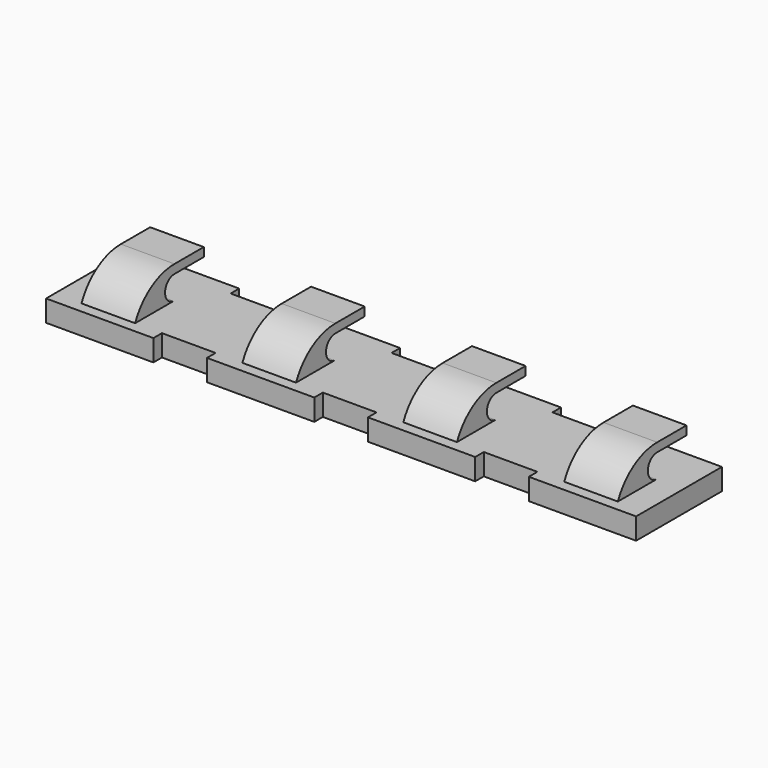
from build123d import *

# Parameters (mm, degrees)
F0_W        = 5
F0_H        = 8
F1_DEPTH    = 2
F2_DEPTH    = 5
F3_T1_DEPTH = 27.9128784748
F3_T3_DEPTH = 27.9128784748
F3_T5_DEPTH = 27.9128784748
F3_T7_DEPTH = 27.9128784748
F5_DEPTH    = 65


# Not quite as in the source:
# - a fillet or chamfer that OpenCascade refuses, or shapes differently, is made with other operations: its cross-section is extruded or revolved along the edge and cut away or added


with BuildPart() as f1:
    # F0 (on Top) → F1 (new body)
    with BuildSketch(Plane.XY):
        Polygon((-17.5, 5), (-27.5, 5), (-27.5, -5), (-17.5, -5), (-17.5, -4), (-17.5, 4), align=None)
        with Locations((-22.5, 0)):
            Rectangle(F0_W, F0_H, mode=Mode.SUBTRACT)
        with Locations((-15, 0)):
            Rectangle(F0_W, F0_H)
        Polygon((-12.5, 5), (-12.5, 4), (-12.5, -4), (-12.5, -5), (-2.5, -5), (-2.5, -4), (-2.5, 4), (-2.5, 5), align=None)
        with Locations((-7.5, 0)):
            Rectangle(F0_W, F0_H, mode=Mode.SUBTRACT)
        Rectangle(F0_W, F0_H)
        Polygon((2.5, 5), (2.5, 4), (2.5, -4), (2.5, -5), (12.5, -5), (12.5, -4), (12.5, 4), (12.5, 5), align=None)
        with Locations((7.5, 0)):
            Rectangle(F0_W, F0_H, mode=Mode.SUBTRACT)
        with Locations((15, 0)):
            Rectangle(F0_W, F0_H)
        Polygon((17.5, 5), (17.5, 4), (17.5, -4), (17.5, -5), (27.5, -5), (27.5, 5), align=None)
        with Locations((22.5, 0)):
            Rectangle(F0_W, F0_H, mode=Mode.SUBTRACT)
    extrude(amount=F1_DEPTH)

    # F0 (on Top) → F2 (join)
    with BuildSketch(Plane.XY):
        with Locations((-22.5, 0)):
            Rectangle(F0_W, F0_H)
        with Locations((-7.5, 0)):
            Rectangle(F0_W, F0_H)
        with Locations((7.5, 0)):
            Rectangle(F0_W, F0_H)
        with Locations((22.5, 0)):
            Rectangle(F0_W, F0_H)
    extrude(amount=F2_DEPTH)

    # F3: fillet of radius 5 on 4 edges, made by hand

    # F3_s2 → F3_t1 (cut)
    with BuildSketch(Plane.YZ.offset(-36.4564392374)):
        with BuildLine():
            ThreePointArc((-4, 2), (-2.1560370926, 4.1833001327), (0.582575695, 5))
            Line((0.582575695, 5), (0.582575695, 5.1))
            Line((0.582575695, 5.1), (-4, 5.1))
            Line((-4, 5.1), (-4.1, 5))
            ThreePointArc((-4.1, 5), (-4.1, 3.5), (-4.0916515139, 2.04))
            Line((-4.0916515139, 2.04), (-4, 2))
        make_face()
    extrude(amount=F3_T1_DEPTH, mode=Mode.SUBTRACT)

    # F3_s4 → F3_t3 (cut)
    with BuildSketch(Plane.YZ.offset(-21.4564392374)):
        with BuildLine():
            ThreePointArc((-4, 2), (-2.1560370926, 4.1833001327), (0.582575695, 5))
            Line((0.582575695, 5), (0.582575695, 5.1))
            Line((0.582575695, 5.1), (-4, 5.1))
            Line((-4, 5.1), (-4.1, 5))
            ThreePointArc((-4.1, 5), (-4.1, 3.5), (-4.0916515139, 2.04))
            Line((-4.0916515139, 2.04), (-4, 2))
        make_face()
    extrude(amount=F3_T3_DEPTH, mode=Mode.SUBTRACT)

    # F3_s6 → F3_t5 (cut)
    with BuildSketch(Plane.YZ.offset(-6.4564392374)):
        with BuildLine():
            ThreePointArc((-4, 2), (-2.1560370926, 4.1833001327), (0.582575695, 5))
            Line((0.582575695, 5), (0.582575695, 5.1))
            Line((0.582575695, 5.1), (-4, 5.1))
            Line((-4, 5.1), (-4.1, 5))
            ThreePointArc((-4.1, 5), (-4.1, 3.5), (-4.0916515139, 2.04))
            Line((-4.0916515139, 2.04), (-4, 2))
        make_face()
    extrude(amount=F3_T5_DEPTH, mode=Mode.SUBTRACT)

    # F3_s8 → F3_t7 (cut)
    with BuildSketch(Plane.YZ.offset(8.5435607626)):
        with BuildLine():
            ThreePointArc((-4, 2), (-2.1560370926, 4.1833001327), (0.582575695, 5))
            Line((0.582575695, 5), (0.582575695, 5.1))
            Line((0.582575695, 5.1), (-4, 5.1))
            Line((-4, 5.1), (-4.1, 5))
            ThreePointArc((-4.1, 5), (-4.1, 3.5), (-4.0916515139, 2.04))
            Line((-4.0916515139, 2.04), (-4, 2))
        make_face()
    extrude(amount=F3_T7_DEPTH, mode=Mode.SUBTRACT)

    # F4 (on face) → F5 (cut)
    with BuildSketch(Plane(origin=(-25, 0, 0), x_dir=(0, -1, 0), z_dir=(-1, 0, 0))):
        with BuildLine():
            Line((-0.582575695, 4.1804881766), (-4, 4.1804881766))
            Line((-4, 4.1804881766), (-4, 2))
            Line((-4, 2), (-0.4667459871, 2))
            ThreePointArc((-0.4667459871, 2), (0.5092055571, 3.1451641031), (-0.582575695, 4.1804881766))
        make_face()
    extrude(amount=-F5_DEPTH, mode=Mode.SUBTRACT)


solid = f1.part
